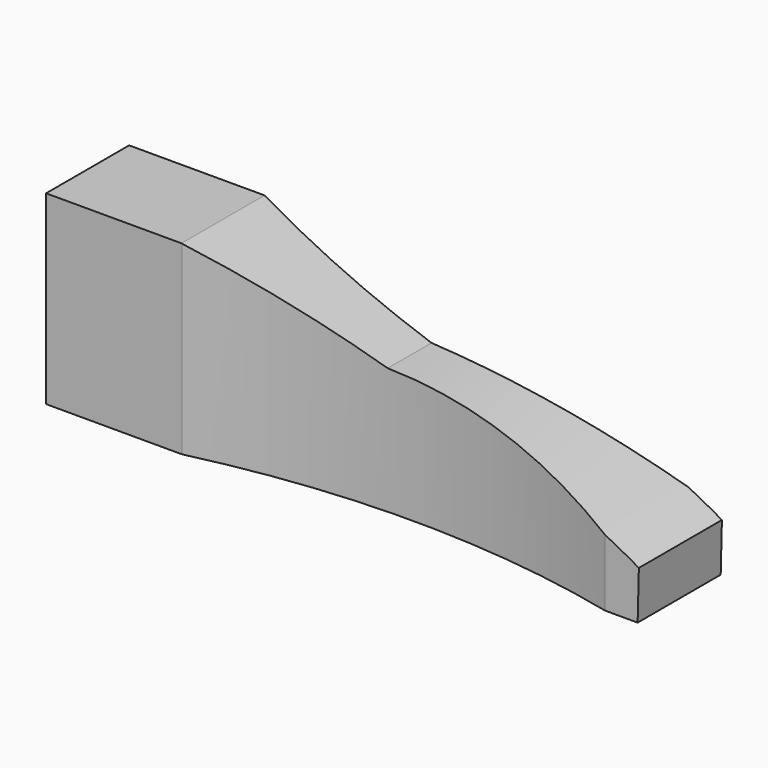
from build123d import *

# Parameters (mm, degrees)
F4_DEPTH = 42
F6_DEPTH = 127
F7_DEPTH = 127
F8_R     = 14.6889125436
F9_DEPTH = 42


# Not quite as in the source:
# - a feature of the source that left no trace in its solid (it failed there, or was rolled back) is left out


with BuildPart() as f4:
    # F2 (on Front) → F4 (new body)
    with BuildSketch(Plane.XZ):
        with BuildLine():
            Line((227.6969850063, 0), (228.1920313835, 19.6573249996))
            ThreePointArc((228.1920313835, 19.6573249996), (175.3476715099, 42.1359663093), (118.6285698173, 51.1225779498))
            Line((118.6285698173, 51.1225779498), (43.1631058455, 75.087800622))
            Line((43.1631058455, 75.087800622), (-11.6123249754, 75.087800622))
            Line((-11.6123249754, 75.087800622), (-11.6123249754, 0))
            Line((-11.6123249754, 0), (227.6969850063, 0))
        make_face()
    extrude(amount=F4_DEPTH)

    # F5 (on face) → F6 (cut)
    with BuildSketch(Plane(origin=(0, 0, 0), x_dir=(1, 0, 0), z_dir=(0, 0, -1))):
        with BuildLine():
            ThreePointArc((214.5471125841, 0), (128.9673938043, 10.0631527668), (43.3876750246, 0))
            Line((43.3876750246, 0), (214.5471125841, 0))
        make_face()
    extrude(amount=-F6_DEPTH, mode=Mode.SUBTRACT)

    # F5 (on face) → F7 (cut)
    with BuildSketch(Plane(origin=(0, 0, 0), x_dir=(1, 0, 0), z_dir=(0, 0, -1))):
        with BuildLine():
            Line((214.5471125841, 42), (43.3876750246, 42))
            ThreePointArc((43.3876750246, 42), (128.9673938043, 31.9368472332), (214.5471125841, 42))
        make_face()
    extrude(amount=-F7_DEPTH, mode=Mode.SUBTRACT)

    # F8 (on face) → F9 (cut)
    with BuildSketch(Plane(origin=(-11.6123249754, 0, 0), x_dir=(0, -1, 0), z_dir=(-1, 0, 0))):
        with Locations((20.4619783908, 53.1766302884)):
            Circle(F8_R)
    extrude(amount=-F9_DEPTH, mode=Mode.SUBTRACT)


solid = f4.part
